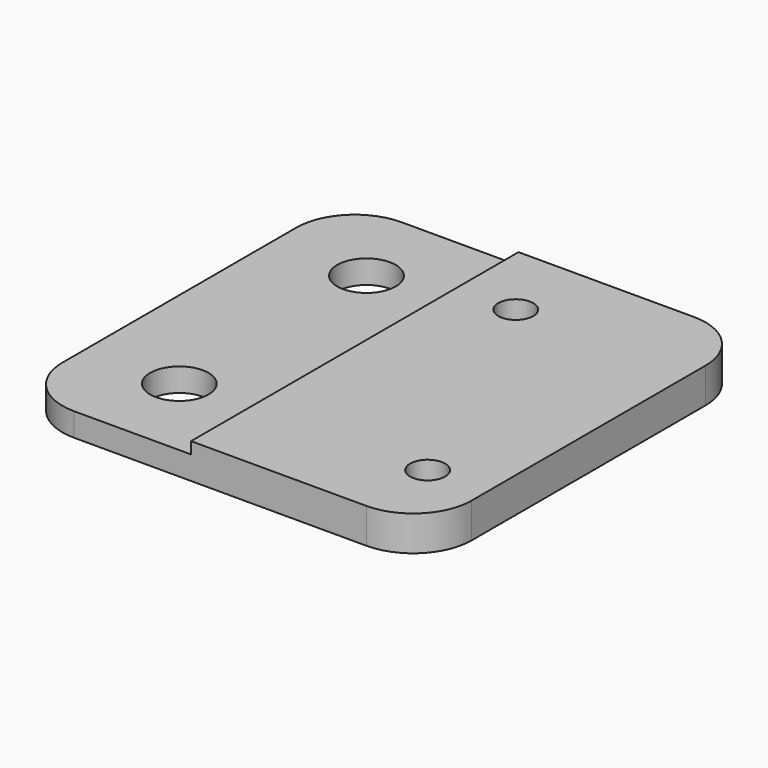
from build123d import *

# Parameters (mm, degrees)
F0_R     = 1.5
F1_DEPTH = 3
F0_R_2   = 2.5
F2_DEPTH = 2


# Not quite as in the source:
# - a feature of the source that left no trace in its solid (it failed there, or was rolled back) is left out


with BuildPart() as f1:
    # F0 (on Top) → F1 (new body)
    with BuildSketch(Plane.XY):
        with BuildLine():
            Line((-2.5, -17.5), (12.5, -17.5))
            ThreePointArc((12.5, -17.5), (16.0355339059, -16.0355339059), (17.5, -12.5))
            Line((17.5, -12.5), (17.5, 12.5))
            ThreePointArc((17.5, 12.5), (16.0355339059, 16.0355339059), (12.5, 17.5))
            Line((12.5, 17.5), (-2.5, 17.5))
            Line((-2.5, 17.5), (-2.5, -17.5))
        make_face()
        with Locations((12.45, -10.9)):
            Circle(F0_R, mode=Mode.SUBTRACT)
        with Locations((2.55, 10.9)):
            Circle(F0_R, mode=Mode.SUBTRACT)
    extrude(amount=F1_DEPTH)

    # F0 (on Top) → F2 (join)
    with BuildSketch(Plane.XY):
        with BuildLine():
            Line((-12.5, -17.5), (-2.5, -17.5))
            Line((-2.5, -17.5), (-2.5, 17.5))
            Line((-2.5, 17.5), (-12.5, 17.5))
            ThreePointArc((-12.5, 17.5), (-16.0355339059, 16.0355339059), (-17.5, 12.5))
            Line((-17.5, 12.5), (-17.5, -12.5))
            ThreePointArc((-17.5, -12.5), (-16.0355339059, -16.0355339059), (-12.5, -17.5))
        make_face()
        with Locations((-9.5, -10)):
            Circle(F0_R_2, mode=Mode.SUBTRACT)
        with Locations((-9.5, 10)):
            Circle(F0_R_2, mode=Mode.SUBTRACT)
    extrude(amount=F2_DEPTH)


solid = f1.part
